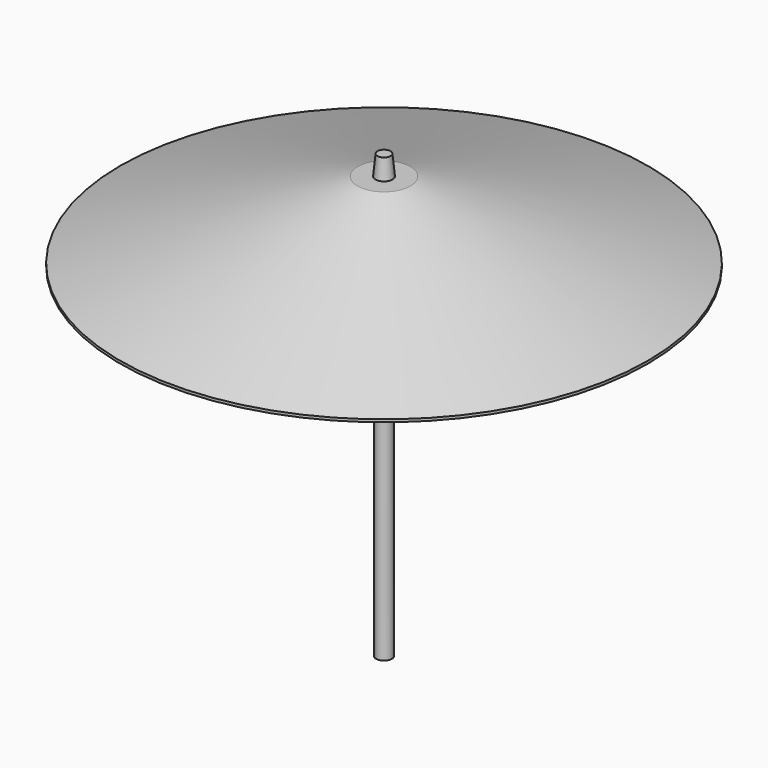
from build123d import *

# Parameters (mm, degrees)
F0_R     = 3
F1_DEPTH = 130
F2_R     = 100
F2_R_2   = 3
F3_DEPTH = 30
F4_SIZE2 = 29
F4_SIZE  = 90
F5_R     = 3.4961547094
F6_DEPTH = 7.6


# Not quite as in the source:
# - a fillet or chamfer that OpenCascade refuses, or shapes differently, is made with other operations: its cross-section is extruded or revolved along the edge and cut away or added


with BuildPart() as f1:
    # F0 (on Top) → F1 (new body)
    with BuildSketch(Plane.XY):
        Circle(F0_R)
    extrude(amount=F1_DEPTH)

    # F2 (on face) → F3 (join)
    with BuildSketch(Plane.XY.offset(130)):
        Circle(F2_R)
        Circle(F2_R_2, mode=Mode.SUBTRACT)
        Circle(F2_R_2)
    extrude(amount=F3_DEPTH)

    # F4
    f4_edges = [f1.edges().sort_by_distance(p)[0] for p in [
        (-100, 0, 160),
    ]]
    f4_side = f1.faces().sort_by_distance((0, 0, 160))[0]
    chamfer(f4_edges, length=F4_SIZE, length2=F4_SIZE2, reference=f4_side)

    # F5 (on face) → F6 (join)
    with BuildSketch(Plane.XY.offset(160)):
        Circle(F5_R)
    extrude(amount=F6_DEPTH)

    # F7: chamfer of 1 x 10 on 1 edges, made by hand


with BuildPart() as f7_tool2:
    # F7_s3 → F7_t4 (revolve)
    with BuildSketch(Plane.XZ):
        Polygon((3.4961547094, 157.6), (2.4961547094, 167.6), (3.4961547094, 167.6), align=None)
    revolve(axis=Axis((0, 0, 167.6), (0, 0, 1)))

    split(bisect_by=Plane.XY.offset(160), keep=Keep.TOP)


with BuildPart() as f1_1:
    add(f1.part)

    # F7_t1: cut F7_tool2
    add(f7_tool2.part, mode=Mode.SUBTRACT)


solid = f1_1.part
